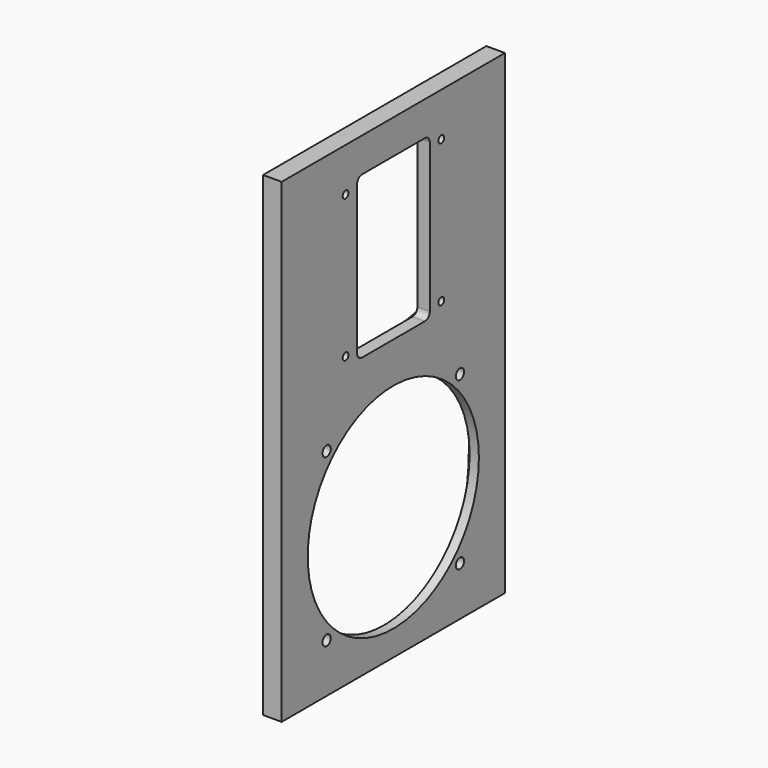
from build123d import *

# Parameters (mm, degrees)
F1_DEPTH = 9
F0_R     = 2.5
F0_R_2   = 51.75
F2_DEPTH = 4.5
F0_R_3   = 3
F0_R_4   = 1.75
F3_R     = 11
F4_DEPTH = 6
F5_R     = 6


# Not quite as in the source:
# - a feature names something its author has since deleted; it is built from what else it names


with BuildPart() as f1:
    # F0 (on Right) → F1 (new body)
    with BuildSketch(Plane.YZ):
        Polygon((67.5, -115), (67.5, 115), (0, 115), (-67.5, 115), (-67.5, -115), align=None)
        with BuildLine():
            ThreePointArc((-47.0226009489, -3.9773990511), (-24.0347326375, 3.4781900517), (0, 6))
            ThreePointArc((0, 6), (24.0347326375, 3.4781900517), (47.0226009489, -3.9773990511))
            ThreePointArc((47.0226009489, -3.9773990511), (57, -51), (47.0226009489, -98.0226009489))
            ThreePointArc((47.0226009489, -98.0226009489), (0, -108), (-47.0226009489, -98.0226009489))
            ThreePointArc((-47.0226009489, -98.0226009489), (-57, -51), (-47.0226009489, -3.9773990511))
        make_face(mode=Mode.SUBTRACT)
        with BuildLine():
            add(Edge.make_bspline(
                [(0, 102.9074018363), (-10.9007532398, 102.8937314348), (-21.8015064796, 100.0876465048), (-32.7022597194, 98.4757185701)],
                knots=[0.5012187781, 0.5012187781, 0.5012187781, 0.5012187781, 1, 1, 1, 1], degree=3))
            add(Edge.make_bspline(
                [(32.8620764687, 98.4757185701), (21.934687104, 100.0915852706), (10.9806616144, 102.9143158042), (0.0266361249, 102.9074352401), (0, 102.9074018363)],
                knots=[0, 0, 0, 0, 0.5, 0.5012187781, 0.5012187781, 0.5012187781, 0.5012187781], degree=3))
            add(Edge.make_bspline(
                [(32.8620764687, 20.339185372), (35.4709924216, 33.361940905), (38.6888243276, 59.4074519711), (35.4709924216, 85.4529630371), (32.8620764687, 98.4757185701)],
                knots=[0, 0, 0, 0, 0.5, 1, 1, 1, 1], degree=3))
            add(Edge.make_bspline(
                [(0, 15.9075021058), (0.0266361249, 15.907468702), (10.9806616144, 15.9005881379), (21.934687104, 18.7233186715), (32.8620764687, 20.339185372)],
                knots=[0.4987812219, 0.4987812219, 0.4987812219, 0.4987812219, 0.5, 1, 1, 1, 1], degree=3))
            add(Edge.make_bspline(
                [(-32.7022597194, 20.339185372), (-21.8015064796, 18.7272574373), (-10.9007532398, 15.9211725073), (0, 15.9075021058)],
                knots=[0, 0, 0, 0, 0.4987812219, 0.4987812219, 0.4987812219, 0.4987812219], degree=3))
            add(Edge.make_bspline(
                [(-32.7022597194, 98.4757185701), (-35.3111756724, 85.4529630371), (-38.5290075784, 59.4074519711), (-35.3111756724, 33.361940905), (-32.7022597194, 20.339185372)],
                knots=[0, 0, 0, 0, 0.5, 1, 1, 1, 1], degree=3))
        make_face(mode=Mode.SUBTRACT)
    extrude(amount=-F1_DEPTH)

    # F0 (on Right) → F2 (join)
    with BuildSketch(Plane.YZ):
        with BuildLine():
            ThreePointArc((47.0226009489, -3.9773990511), (24.0347326375, 3.4781900517), (0, 6))
            ThreePointArc((0, 6), (-24.0347326375, 3.4781900517), (-47.0226009489, -3.9773990511))
            ThreePointArc((-47.0226009489, -3.9773990511), (-57, -51), (-47.0226009489, -98.0226009489))
            ThreePointArc((-47.0226009489, -98.0226009489), (0, -108), (47.0226009489, -98.0226009489))
            ThreePointArc((47.0226009489, -98.0226009489), (57, -51), (47.0226009489, -3.9773990511))
        make_face()
        with Locations((-40.3050865276, -91.3050865276)):
            Circle(F0_R, mode=Mode.SUBTRACT)
        with Locations((-40.3050865276, -10.6949134724)):
            Circle(F0_R, mode=Mode.SUBTRACT)
        with Locations((40.3050865276, -91.3050865276)):
            Circle(F0_R, mode=Mode.SUBTRACT)
        with Locations((0, -51)):
            Circle(F0_R_2, mode=Mode.SUBTRACT)
        with Locations((40.3050865276, -10.6949134724)):
            Circle(F0_R, mode=Mode.SUBTRACT)
    extrude(amount=-F2_DEPTH)

    # F3
    f3_edges = [f1.edges().sort_by_distance(p)[0] for p in [
        (-6.75, 47.022601, -3.977399),
        (-6.75, -47.022601, -3.977399),
        (-6.75, -47.022601, -98.022601),
        (-6.75, 47.022601, -98.022601),
    ]]
    fillet(f3_edges, radius=F3_R)



with BuildPart() as f2:
    # F0 (on Right) → F2, piece 2 (new body)
    with BuildSketch(Plane.YZ):
        with Locations((-28.8455340613, 24.9354520307)):
            Circle(F0_R_3)
        with Locations((-28.8455340613, 24.9354520307)):
            Circle(F0_R_4, mode=Mode.SUBTRACT)
    extrude(amount=-F2_DEPTH)


with BuildPart() as f2b:
    # F0 (on Right) → F2, piece 3 (new body)
    with BuildSketch(Plane.YZ):
        with Locations((29.0053508105, 24.9354520307)):
            Circle(F0_R_3)
        with Locations((29.0053508105, 24.9354520307)):
            Circle(F0_R_4, mode=Mode.SUBTRACT)
    extrude(amount=-F2_DEPTH)


with BuildPart() as f1_1:
    add(f1.part)

    add(f2.part)  # F4 merges F2

    add(f2b.part)  # F4 merges F2b
    # F0 (on Right) → F4 (join)
    with BuildSketch(Plane.YZ):
        with BuildLine():
            add(Edge.make_bspline(
                [(32.8620764687, 98.4757185701), (21.934687104, 100.0915852706), (10.9806616144, 102.9143158042), (0.0266361249, 102.9074352401), (0, 102.9074018363)],
                knots=[0, 0, 0, 0, 0.5, 0.5012187781, 0.5012187781, 0.5012187781, 0.5012187781], degree=3))
            Line((0, 102.9074018363), (0, 98.4074519711))
            Line((0, 98.4074519711), (19.0799083746, 98.4074519711))
            ThreePointArc((19.0799083746, 98.4074519711), (21.2012287182, 97.5287723146), (22.0799083746, 95.4074519711))
            Line((22.0799083746, 95.4074519711), (22.0799083746, 23.4074519711))
            ThreePointArc((22.0799083746, 23.4074519711), (21.2012287182, 21.2861316275), (19.0799083746, 20.4074519711))
            Line((19.0799083746, 20.4074519711), (0, 20.4074519711))
            Line((0, 20.4074519711), (0, 15.9075021058))
            add(Edge.make_bspline(
                [(0, 15.9075021058), (0.0266361249, 15.907468702), (10.9806616144, 15.9005881379), (21.934687104, 18.7233186715), (32.8620764687, 20.339185372)],
                knots=[0.4987812219, 0.4987812219, 0.4987812219, 0.4987812219, 0.5, 1, 1, 1, 1], degree=3))
            add(Edge.make_bspline(
                [(32.8620764687, 20.339185372), (35.4709924216, 33.361940905), (38.6888243276, 59.4074519711), (35.4709924216, 85.4529630371), (32.8620764687, 98.4757185701)],
                knots=[0, 0, 0, 0, 0.5, 1, 1, 1, 1], degree=3))
        make_face()
        with Locations((29.0053508105, 24.9354520307)):
            Circle(F0_R_3, mode=Mode.SUBTRACT)
        with Locations((29.0053508105, 93.8794519114)):
            Circle(F0_R_3, mode=Mode.SUBTRACT)
        with BuildLine():
            Line((0, 98.4074519711), (0, 102.9074018363))
            add(Edge.make_bspline(
                [(0, 102.9074018363), (-10.9007532398, 102.8937314348), (-21.8015064796, 100.0876465048), (-32.7022597194, 98.4757185701)],
                knots=[0.5012187781, 0.5012187781, 0.5012187781, 0.5012187781, 1, 1, 1, 1], degree=3))
            add(Edge.make_bspline(
                [(-32.7022597194, 98.4757185701), (-35.3111756724, 85.4529630371), (-38.5290075784, 59.4074519711), (-35.3111756724, 33.361940905), (-32.7022597194, 20.339185372)],
                knots=[0, 0, 0, 0, 0.5, 1, 1, 1, 1], degree=3))
            add(Edge.make_bspline(
                [(-32.7022597194, 20.339185372), (-21.8015064796, 18.7272574373), (-10.9007532398, 15.9211725073), (0, 15.9075021058)],
                knots=[0, 0, 0, 0, 0.4987812219, 0.4987812219, 0.4987812219, 0.4987812219], degree=3))
            Line((0, 15.9075021058), (0, 20.4074519711))
            Line((0, 20.4074519711), (-18.9200916254, 20.4074519711))
            ThreePointArc((-18.9200916254, 20.4074519711), (-21.0414119689, 21.2861316275), (-21.9200916254, 23.4074519711))
            Line((-21.9200916254, 23.4074519711), (-21.9200916254, 95.4074519711))
            ThreePointArc((-21.9200916254, 95.4074519711), (-21.0414119689, 97.5287723146), (-18.9200916254, 98.4074519711))
            Line((-18.9200916254, 98.4074519711), (0, 98.4074519711))
        make_face()
        with Locations((-28.8455340613, 24.9354520307)):
            Circle(F0_R_3, mode=Mode.SUBTRACT)
        with Locations((-28.8455340613, 93.8794519114)):
            Circle(F0_R_3, mode=Mode.SUBTRACT)
        with Locations((29.0053508105, 93.8794519114)):
            Circle(F0_R_3)
        with Locations((29.0053508105, 93.8794519114)):
            Circle(F0_R_4, mode=Mode.SUBTRACT)
        with Locations((-28.8455340613, 93.8794519114)):
            Circle(F0_R_3)
        with Locations((-28.8455340613, 93.8794519114)):
            Circle(F0_R_4, mode=Mode.SUBTRACT)
        with Locations((-28.8455340613, 24.9354520307)):
            Circle(F0_R_3)
        with Locations((-28.8455340613, 24.9354520307)):
            Circle(F0_R_4, mode=Mode.SUBTRACT)
        with Locations((29.0053508105, 24.9354520307)):
            Circle(F0_R_3)
        with Locations((29.0053508105, 24.9354520307)):
            Circle(F0_R_4, mode=Mode.SUBTRACT)
    extrude(amount=-F4_DEPTH)

    # F5
    f5_edges = [f1_1.edges().sort_by_distance(p)[0] for p in [
        (-7.5, 32.862076, 98.475719),
        (-7.5, 32.862076, 20.339185),
        (-7.5, -32.70226, 20.339185),
        (-7.5, -32.70226, 98.475719),
    ]]
    fillet(f5_edges, radius=F5_R)


solid = f1_1.part
